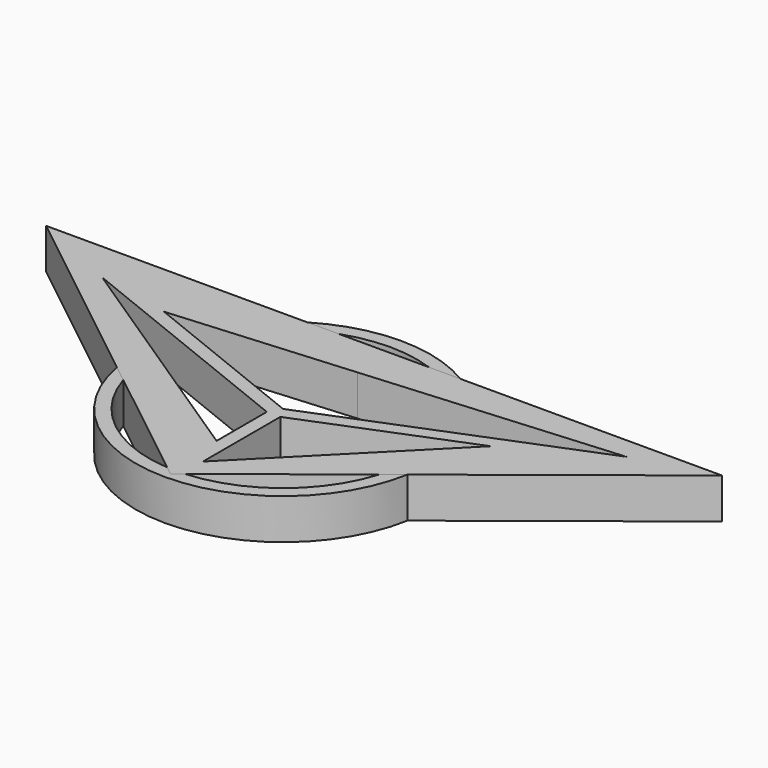
from build123d import *

# Parameters (mm, degrees)
F1_DEPTH = 3
F2_DEPTH = 3
F3_DEPTH = 3


# Not quite as in the source:
# - a feature names something its author has since deleted; it is built from what else it names


with BuildPart() as f1:
    # F0 (on Top) → F1 (new body)
    with BuildSketch(Plane.XY):
        Polygon((3.3342897613, 0), (0, 0), (-3.3342897613, 0), (-5.6521106464, 0), (-25, 0), (-10.7429983194, -11.263816016), (-9.4710395464, -12.2687334537), (-0.6607687547, -19.2293322859), (0, -19.7513759701), (0.6607687547, -19.2293322859), (9.4710395464, -12.2687334537), (10.7429983194, -11.263816016), (25, 0), (5.6521106464, 0), align=None)
        Polygon((-20.7355933027, -2.094680059), (-22.1211677314, -1), (-20.7784352121, -1), (0, -1), (14.3438164741, -1), (20.7784352121, -1), (22.1211677314, -1), (20.7355933027, -2.094680059), (3.7483545568, -15.5155336256), (0.5, -18.081912511), (0, -18.4769400304), (-0.5, -18.081912511), (-16.112200225, -5.7474150564), align=None, mode=Mode.SUBTRACT)
        Polygon((0.5, -17.3717289222), (0.5, -18.081912511), (3.7483545568, -15.5155336256), (14.6217098136, -4.5477568082), (12.2834767919, -5.4859272967), align=None)
        Polygon((-0.5, -16.0585195866), (-0.5, -18.081912511), (0, -18.4769400304), (0.5, -18.081912511), (0.5, -17.3717289222), (0.5, -10.2138180054), (0.5, -9.1363274287), (0, -9.3369426967), (-0.5, -9.1363274287), (-0.5, -10.2138180054), (-0.5, -14.8601054354), align=None)
        Polygon((22.1211677314, -1), (20.7784352121, -1), (19.2271466743, -1.6224243315), (0.5, -9.1363274287), (0.5, -10.2138180054), (12.2834767919, -5.4859272967), (14.6217098136, -4.5477568082), (20.7355933027, -2.094680059), align=None)
        Polygon((20.7784352121, -1), (14.3438164741, -1), (0.5, -2.0789917684), (0.5, -3.0820245179), (19.2271466743, -1.6224243315), align=None)
        Polygon((0.5, -2.0789917684), (-0.5, -2.1569321088), (-0.5, -3.1599648583), (0.5, -3.0820245179), align=None)
        Polygon((-0.5, -2.1569321088), (-15.0655666155, -3.2921773289), (-12.9722992677, -4.1320601088), (-0.5, -3.1599648583), align=None)
        Polygon((-20.7784352121, -1), (-22.1211677314, -1), (-20.7355933027, -2.094680059), (-18.4240265529, -3.022151225), (-0.5, -10.2138180054), (-0.5, -9.1363274287), (-12.9722992677, -4.1320601088), (-15.0655666155, -3.2921773289), align=None)
        Polygon((-18.4240265529, -3.022151225), (-20.7355933027, -2.094680059), (-16.112200225, -5.7474150564), (-0.5, -16.0585195866), (-0.5, -14.8601054354), align=None)
    extrude(amount=F1_DEPTH)

    # F0 (on Top) → F2 (join)
    with BuildSketch(Plane.XY):
        Polygon((0, -1), (-20.7784352121, -1), (-15.0655666155, -3.2921773289), (-0.5, -2.1569321088), (0.5, -2.0789917684), (14.3438164741, -1), align=None)
        Polygon((3.7483545568, -15.5155336256), (20.7355933027, -2.094680059), (14.6217098136, -4.5477568082), align=None)
        Polygon((-0.5, -16.0585195866), (-16.112200225, -5.7474150564), (-0.5, -18.081912511), align=None)
    extrude(amount=F2_DEPTH)


with BuildPart() as f3:
    # F0 (on Top) → F3 (new body)
    with BuildSketch(Plane.XY):
        with BuildLine():
            ThreePointArc((-3.3342897613, 0), (0, 0.5774905768), (3.3342897613, 0))
            Line((3.3342897613, 0), (5.6521106464, 0))
            ThreePointArc((5.6521106464, 0), (0, 1.5774905768), (-5.6521106464, 0))
            Line((-5.6521106464, 0), (-3.3342897613, 0))
        make_face()
    extrude(amount=F3_DEPTH)


with BuildPart() as f3b:
    # F0 (on Top) → F3, piece 2 (new body)
    with BuildSketch(Plane.XY):
        with BuildLine():
            ThreePointArc((-10.7429983194, -11.263816016), (0, -20.2513759701), (10.7429983194, -11.263816016))
            Line((10.7429983194, -11.263816016), (9.4710395464, -12.2687334537))
            ThreePointArc((9.4710395464, -12.2687334537), (6.1462076835, -17.116410432), (0.6607687547, -19.2293322859))
            Line((0.6607687547, -19.2293322859), (0, -19.7513759701))
            Line((0, -19.7513759701), (-0.6607687547, -19.2293322859))
            ThreePointArc((-0.6607687547, -19.2293322859), (-6.1462076835, -17.116410432), (-9.4710395464, -12.2687334537))
            Line((-9.4710395464, -12.2687334537), (-10.7429983194, -11.263816016))
        make_face()
    extrude(amount=F3_DEPTH)


solid = Compound([f1.part, f3.part, f3b.part])
